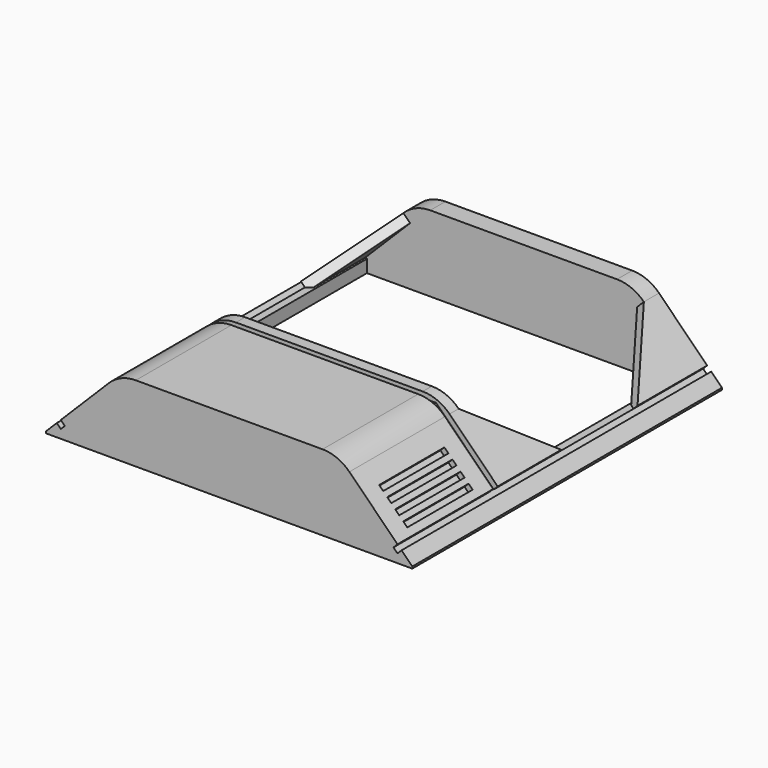
from build123d import *

# Parameters (mm, degrees)
F1_DEPTH  = 20.4
F3_DEPTH  = 0.3
F4_W      = 12.2
F4_H      = 3.3343145751
F5_DEPTH  = 8.8731825407
F6_W      = 8.2600505063
F6_H      = 12.2
F7_DEPTH  = 25
F8_W      = 4.3
F8_H      = 0.3
F9_DEPTH  = 0.3
F10_F1_R  = 2
F10_F2_R  = 2
F12_DEPTH = 0.5
F13_W     = 8.8721825407
F13_H     = 0.3
F14_DEPTH = 0.3
F16_DEPTH = 0.1


# Not quite as in the source:
# - a feature names something its author has since deleted; it is built from what else it names


with BuildPart() as f1:
    # F0 (on Front) → F1 (new body)
    with BuildSketch(Plane.XZ):
        Polygon((-9.65, 0), (0, 0), (0, 3.9), (-5.75, 3.9), align=None)
    extrude(amount=F1_DEPTH)

    # F2 (on face) → F3 (cut)
    with BuildSketch(Plane(origin=(-4.825, 0, 4.825), x_dir=(0, -1, 0), z_dir=(-0.7071067812, 0, 0.7071067812))):
        Polygon((13.8, -5.7235804385), (0, -5.7235804385), (0, -6.0235804385), (20.4, -6.0235804385), (20.4, -5.7235804385), (14.1, -5.7235804385), (14.1, 0.1956567054), (13.8, 0.1956567054), align=None)
    extrude(amount=-F3_DEPTH, mode=Mode.SUBTRACT)

    # F4 (on face) → F5 (cut, through all)
    with BuildSketch(Plane.YZ):
        with Locations((-7.1, 2.2328427125)):
            Rectangle(F4_W, F4_H)
    extrude(amount=-F5_DEPTH, mode=Mode.SUBTRACT)

    # F6 (on face) → F7 (cut)
    with BuildSketch(Plane.XY.offset(0.5656854249)):
        with Locations((-4.1300252532, -7.1)):
            Rectangle(F6_W, F6_H)
    extrude(amount=-F7_DEPTH, mode=Mode.SUBTRACT)

    # F8 (on face) → F9 (cut)
    with BuildSketch(Plane(origin=(-4.825, 0, 4.825), x_dir=(0, -1, 0), z_dir=(-0.7071067812, 0, 0.7071067812))):
        with Locations((17.25, -3.3735804385)):
            Rectangle(F8_W, F8_H)
        with Locations((17.25, -3.9735804385)):
            Rectangle(F8_W, F8_H)
        with Locations((17.25, -5.1735804385)):
            Rectangle(F8_W, F8_H)
        with Locations((17.25, -4.5735804385)):
            Rectangle(F8_W, F8_H)
    extrude(amount=-F9_DEPTH, mode=Mode.SUBTRACT)

    # F10: fillet of radius 2 on 3 edges, made by hand

    # F10_f1
    f10_f1_edges = [f1.edges().sort_by_distance(p)[0] for p in [
        (-5.75, -0.5, 3.9),
    ]]
    fillet(f10_f1_edges, radius=F10_F1_R)

    # F10_f2
    f10_f2_edges = [f1.edges().sort_by_distance(p)[0] for p in [
        (-5.75, -13.5, 3.9),
    ]]
    fillet(f10_f2_edges, radius=F10_F2_R)

    # F11 (on face) → F12 (join)
    with BuildSketch(Plane(origin=(-4.825, 0, 4.825), x_dir=(0, -1, 0), z_dir=(-0.7071067812, 0, 0.7071067812))):
        Polygon((1, -2.1365746699), (1, -5.7235804385), (4.5870057685, -5.7235804385), align=None)
        Polygon((13.2, -5.7235804385), (13.2, -2.1365746699), (9.6129942315, -5.7235804385), align=None)
    extrude(amount=-F12_DEPTH)

    # F13 (on face) → F14 (cut)
    with BuildSketch(Plane.XY.offset(3.9)):
        with Locations((-4.4360912703, -13.95)):
            Rectangle(F13_W, F13_H)
    extrude(amount=-F14_DEPTH, mode=Mode.SUBTRACT)

    # F15: F1 across face


with BuildPart() as f1_1:
    add(f1.part)
    add(f1.part.mirror(Plane(origin=(0, -16.8091639871, 1.9442122186), x_dir=(0, 1, 0), z_dir=(1, 0, 0))))

    # F16 (add): a face of the model
    f16_faces = [f1_1.faces().sort_by_distance(p)[0] for p in [
        (0, -13.4511563716, 0),
    ]]
    extrude(f16_faces, amount=F16_DEPTH)


solid = f1_1.part
